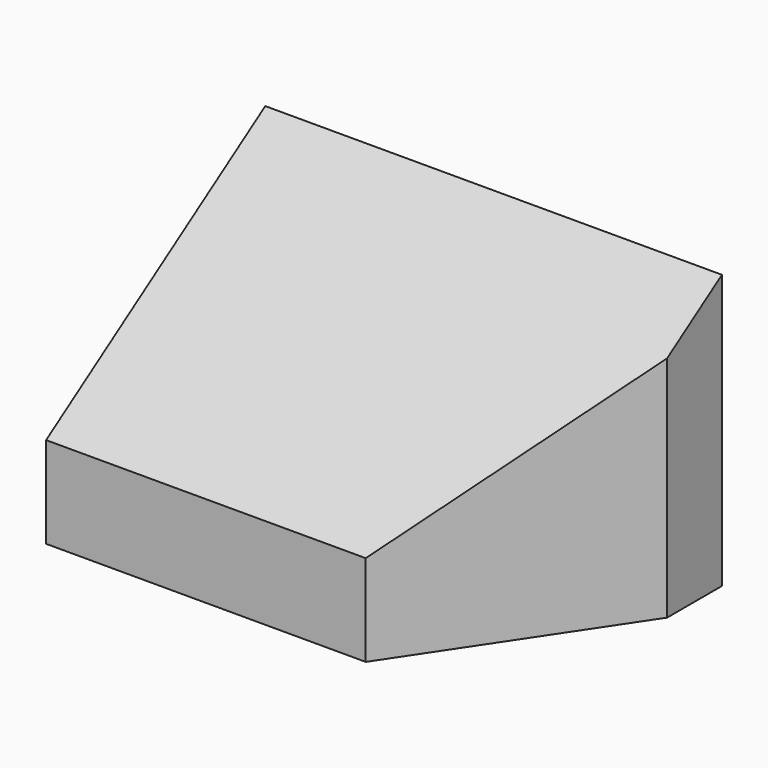
from build123d import *

# Parameters (mm, degrees)
F0_W     = 100
F0_H     = 60
F1_DEPTH = 60
F4_DEPTH = 60.001
F5_DEPTH = 100.001


# Not quite as in the source:
# - a feature names something its author has since deleted; it is built from what else it names


with BuildPart() as f1:
    # F0 (on Front) → F1 (new body)
    with BuildSketch(Plane.XZ):
        with Locations((50, 30)):
            Rectangle(F0_W, F0_H)
    extrude(amount=F1_DEPTH)

    # F3 (on face) → F4 (cut, through all)
    with BuildSketch(Plane.XY.offset(60)):
        Polygon((100, -60), (100, -15), (70, -60), align=None)
    extrude(amount=-F4_DEPTH, mode=Mode.SUBTRACT)

    # F2 (on face) → F5 (cut, through all)
    with BuildSketch(Plane(origin=(0, 0, 0), x_dir=(0, -1, 0), z_dir=(-1, 0, 0))):
        Polygon((60, 60), (0, 60), (60, 20), align=None)
    extrude(amount=-F5_DEPTH, mode=Mode.SUBTRACT)


solid = f1.part
